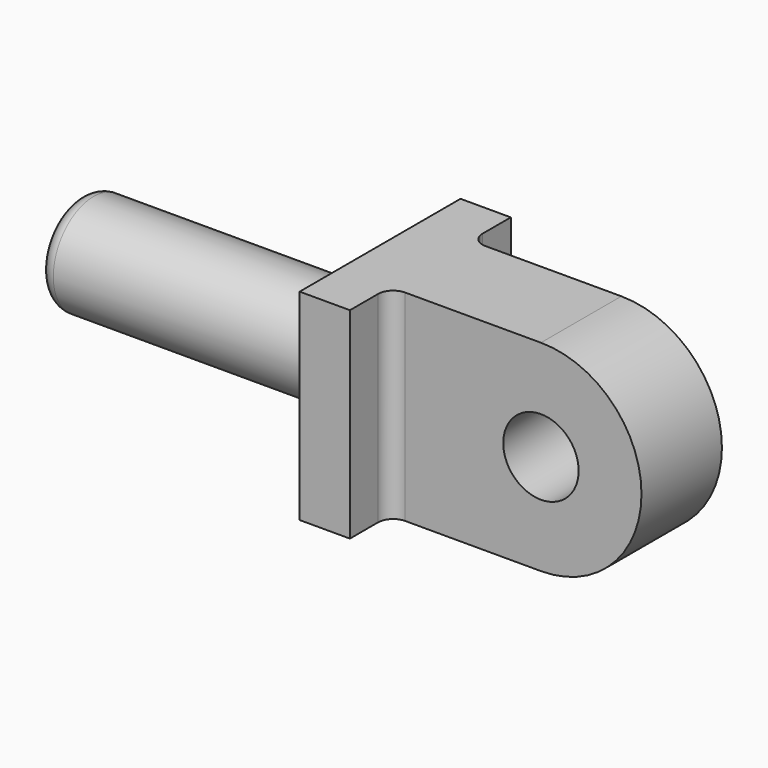
from build123d import *

# Parameters (mm, degrees)
F0_W     = 50.8
F0_H     = 50.8
F1_DEPTH = 12.7
F2_R     = 12.7
F3_DEPTH = 76.2
F4_R     = 9.525
F5_DEPTH = 38.1
F6_DEPTH = 12.7
F7_R     = 3.81


with BuildPart() as f1:
    # F0 (on Right) → F1 (new body)
    with BuildSketch(Plane.YZ):
        Rectangle(F0_W, F0_H)
    extrude(amount=F1_DEPTH)

    # F2 (on face) → F3 (join)
    with BuildSketch(Plane(origin=(0, 0, 0), x_dir=(0, -1, 0), z_dir=(-1, 0, 0))):
        Circle(F2_R)
    extrude(amount=F3_DEPTH)

    # F4 (on face) → F5 (join)
    with BuildSketch(Plane.XZ.offset(25.4)):
        with BuildLine():
            Line((50.8, 25.4), (12.7, 25.4))
            Line((12.7, 25.4), (12.7, -25.4))
            Line((12.7, -25.4), (50.8, -25.4))
            ThreePointArc((50.8, -25.4), (76.2, 0), (50.8, 25.4))
        make_face()
        with Locations((50.8, 0)):
            Circle(F4_R, mode=Mode.SUBTRACT)
    extrude(amount=-F5_DEPTH)

    # F4 (on face) → F6 (cut)
    with BuildSketch(Plane.XZ.offset(25.4)):
        with BuildLine():
            Line((50.8, 25.4), (12.7, 25.4))
            Line((12.7, 25.4), (12.7, -25.4))
            Line((12.7, -25.4), (50.8, -25.4))
            ThreePointArc((50.8, -25.4), (76.2, 0), (50.8, 25.4))
        make_face()
        with Locations((50.8, 0)):
            Circle(F4_R, mode=Mode.SUBTRACT)
    extrude(amount=-F6_DEPTH, mode=Mode.SUBTRACT)

    # F7
    f7_edges = [f1.edges().sort_by_distance(p)[0] for p in [
        (-76.2, 12.7, 0),
        (0, 12.7, 0),
        (12.7, -12.7, 0),
        (12.7, 12.7, 0),
    ]]
    fillet(f7_edges, radius=F7_R)


solid = f1.part
